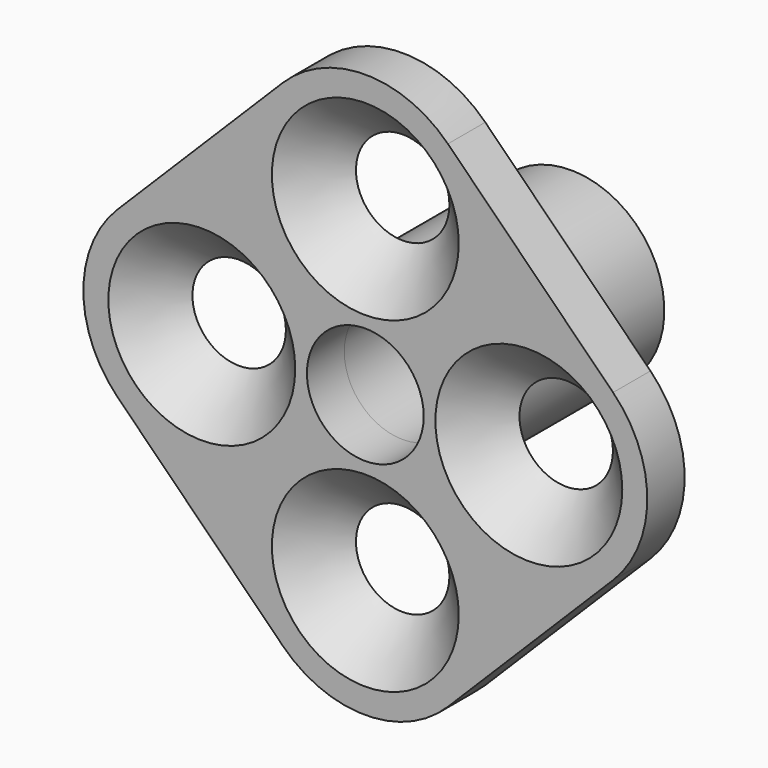
from build123d import *

# Parameters (mm, degrees)
F0_R     = 2
F0_R_2   = 2.5
F1_DEPTH = 2
F2_SIZE  = 1.99999
F3_R     = 4
F3_R_2   = 2.5
F4_DEPTH = 9


# Not quite as in the source:
# - a fillet or chamfer is up to 0.001 mm smaller than in the source, because OpenCascade refuses the exact size


with BuildPart() as f1:
    # F0 (on Front) → F1 (new body)
    with BuildSketch(Plane.XZ):
        with BuildLine():
            Line((-10.6066017178, -3.5355339059), (-3.5355339059, -10.6066017178))
            ThreePointArc((-3.5355339059, -10.6066017178), (0, -12.0710678119), (3.5355339059, -10.6066017178))
            Line((3.5355339059, -10.6066017178), (10.6066017178, -3.5355339059))
            ThreePointArc((10.6066017178, -3.5355339059), (12.0710678119, 0), (10.6066017178, 3.5355339059))
            Line((10.6066017178, 3.5355339059), (3.5355339059, 10.6066017178))
            ThreePointArc((3.5355339059, 10.6066017178), (0, 12.0710678119), (-3.5355339059, 10.6066017178))
            Line((-3.5355339059, 10.6066017178), (-10.6066017178, 3.5355339059))
            ThreePointArc((-10.6066017178, 3.5355339059), (-12.0710678119, 0), (-10.6066017178, -3.5355339059))
        make_face()
        with Locations((-7, 0)):
            Circle(F0_R, mode=Mode.SUBTRACT)
        with Locations((0, -7)):
            Circle(F0_R, mode=Mode.SUBTRACT)
        Circle(F0_R_2, mode=Mode.SUBTRACT)
        with Locations((7, 0)):
            Circle(F0_R, mode=Mode.SUBTRACT)
        with Locations((0, 7)):
            Circle(F0_R, mode=Mode.SUBTRACT)
    extrude(amount=F1_DEPTH)

    # F2 (size 2 in the source; OpenCascade refuses exactly that, so slightly less here)
    f2_edges = [f1.edges().sort_by_distance(p)[0] for p in [
        (5, -2, 0),
        (-2, -2, -7),
        (-9, -2, 0),
        (-2, -2, 7),
    ]]
    chamfer(f2_edges, length=F2_SIZE)

    # F3 (on face) → F4 (join)
    with BuildSketch(Plane(origin=(0, 0, 0), x_dir=(-1, 0, 0), z_dir=(0, 1, 0))):
        Circle(F3_R)
        Circle(F3_R_2, mode=Mode.SUBTRACT)
    extrude(amount=F4_DEPTH)


solid = f1.part
